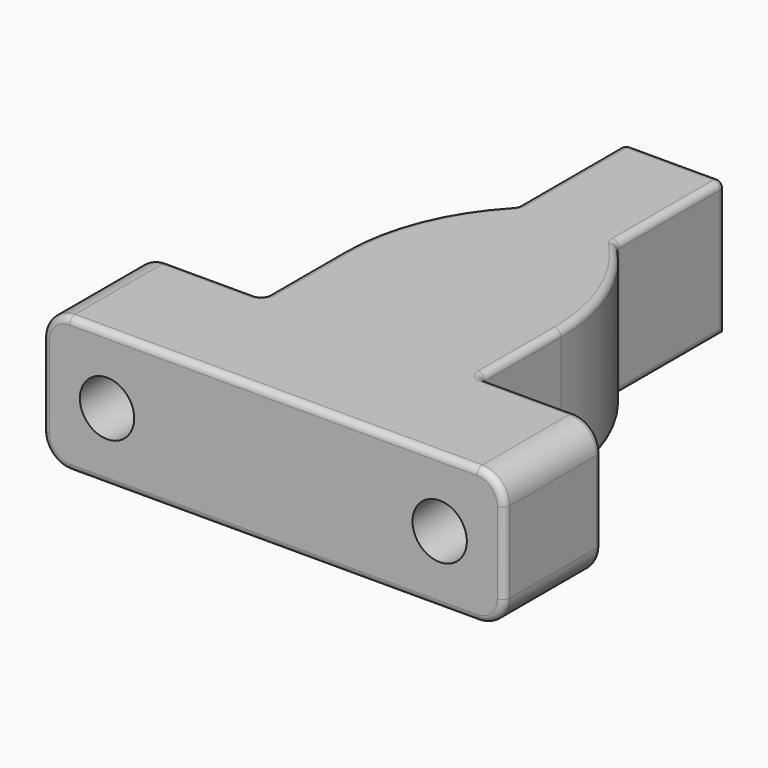
from build123d import *

# Parameters (mm, degrees)
F0_W           = 9
F0_H           = 10
F0_W_2         = 4.3
F0_W_3         = 7.4
F1_DEPTH       = 9
F2_D           = 4
F2_DEPTH       = 12
F2_CBORE_D     = 6.5
F2_CBORE_DEPTH = 3
F2_TIP         = 1.2017212381
F3_DEPTH       = 18
F4_DEPTH       = 28
F5_T1_DEPTH    = 62.5618683077
F6_R           = 2
F7_R           = 0.5


# Not quite as in the source:
# - a fillet or chamfer that OpenCascade refuses, or shapes differently, is made with other operations: its cross-section is extruded or revolved along the edge and cut away or added


with BuildPart() as f1:
    # F0 (on Front) → F1 (new body)
    with BuildSketch(Plane.XZ):
        with Locations((-4.5, 5)):
            Rectangle(F0_W, F0_H)
        with Locations((-11.15, 5)):
            Rectangle(F0_W_2, F0_H)
        with Locations((-17, 5)):
            Rectangle(F0_W_3, F0_H)
        with Locations((-22.85, 5)):
            Rectangle(F0_W_2, F0_H)
        with Locations((-29.5, 5)):
            Rectangle(F0_W, F0_H)
    extrude(amount=F1_DEPTH)

    # F2
    with Locations(Plane(origin=(0, 0, 0), x_dir=(1, 0, 0), z_dir=(0, 1, 0))):
        with Locations((-29.25, -5), (-4.75, -5)):
            CounterBoreHole(F2_D / 2, F2_CBORE_D / 2, F2_CBORE_DEPTH, depth=F2_DEPTH)
            with Locations((0, 0, -(F2_DEPTH + F2_TIP / 2))):  # 118° drill point
                Cone(0, F2_D / 2, F2_TIP, mode=Mode.SUBTRACT)

    # F0 (on Front) → F3 (join)
    with BuildSketch(Plane.XZ):
        with Locations((-22.85, 5)):
            Rectangle(F0_W_2, F0_H)
        with Locations((-17, 5)):
            Rectangle(F0_W_3, F0_H)
        with Locations((-11.15, 5)):
            Rectangle(F0_W_2, F0_H)
    extrude(amount=-F3_DEPTH)

    # F0 (on Front) → F4 (join)
    with BuildSketch(Plane.XZ):
        with Locations((-17, 5)):
            Rectangle(F0_W_3, F0_H)
    extrude(amount=-F4_DEPTH)

    # F5: fillet of radius 15 on 2 edges, made by hand

    # F5_s2 → F5_t1 (cut)
    with BuildSketch(Plane.XY.offset(-26.2809341539)):
        with BuildLine():
            ThreePointArc((-13.3, 18), (-10.1165566231, 13.1665346843), (-9, 7.4876263385))
            Line((-9, 7.4876263385), (-9, 18))
            Line((-9, 18), (-13.3, 18))
        make_face()
        with BuildLine():
            ThreePointArc((-25, 7.4876263385), (-23.8834433769, 13.1665346843), (-20.7, 18))
            Line((-20.7, 18), (-25, 18))
            Line((-25, 18), (-25, 7.4876263385))
        make_face()
    extrude(amount=F5_T1_DEPTH, mode=Mode.SUBTRACT)

    # F6
    f6_edges = [f1.edges().sort_by_distance(p)[0] for p in [
        (0, -4.5, 10),
        (0, -4.5, 0),
        (-34, -4.5, 0),
        (-34, -4.5, 10),
    ]]
    fillet(f6_edges, radius=F6_R)

    # F7
    f7_edges = [f1.edges().sort_by_distance(p)[0] for p in [
        (-9, 0, 5),
        (-25, 0, 5),
        (-25, 7.487626, 5),
        (-20.7, 18, 5),
        (-13.3, 18, 5),
        (-13.3, 28, 5),
        (-20.7, 28, 5),
        (-17, 28, 10),
        (-20.7, 23, 10),
        (-10.116557, 13.166535, 10),
        (-17, -9, 10),
        (0, 0, 5),
        (0, -9, 5),
        (-5.5, 0, 0),
        (-0.585786, 0, 0.585786),
        (-5.5, 0, 10),
        (-0.585786, 0, 9.414214),
        (-0.585786, -9, 0.585786),
        (-0.585786, -9, 9.414214),
        (-17, -9, 0),
        (-33.414214, -9, 0.585786),
        (-33.414214, -9, 9.414214),
        (-34, -9, 5),
        (-28.5, 0, 0),
        (-25, 3.743813, 0),
        (-23.883443, 13.166535, 0),
        (-20.7, 23, 0),
        (-9, 3.743813, 0),
        (-13.3, 23, 0),
        (-10.116557, 13.166535, 0),
        (-9, 3.743813, 10),
        (-13.3, 23, 10),
        (-28.5, 0, 10),
        (-25, 3.743813, 10),
        (-23.883443, 13.166535, 10),
        (-33.414214, 0, 0.585786),
        (-33.414214, 0, 9.414214),
        (-34, 0, 5),
    ]]
    fillet(f7_edges, radius=F7_R)


solid = f1.part
